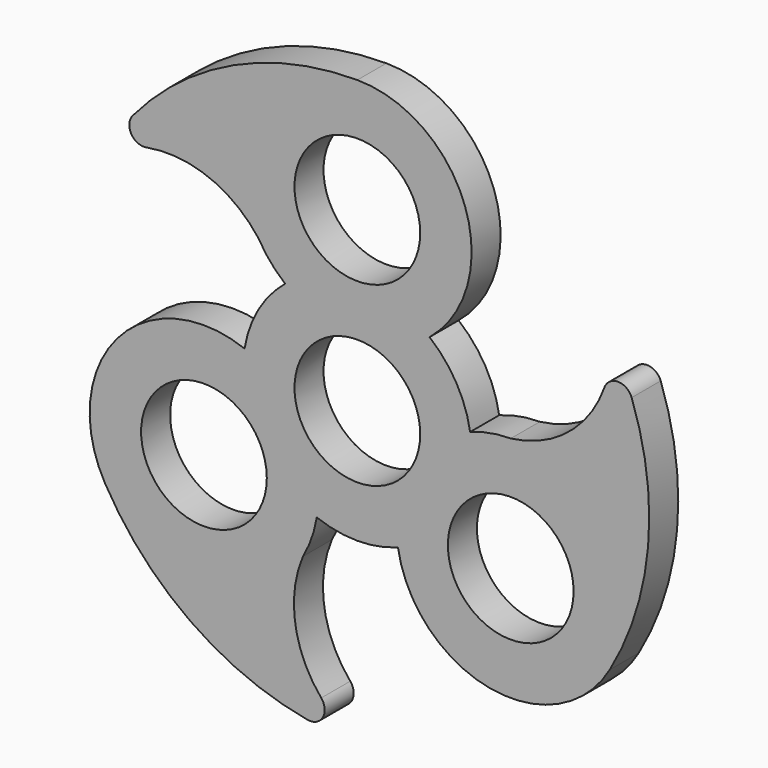
from build123d import *

# Parameters (mm, degrees)
F1_R     = 11
F2_DEPTH = 3.175
F3_COUNT = 3


# Not quite as in the source:
# - a length typed as a fraction of an inch, garbled in the dataset ("3 / 203.2 mm" for 3/8 in), is restored
# - a feature names something its author has since deleted; it is built from what else it names


with BuildPart() as f2:
    # F1 (on Front) → F2 (new body, symmetric)
    with BuildSketch(Plane.XZ):
        with BuildLine():
            ThreePointArc((-17.3205080757, 21), (-15.23019686, 18.0369330942), (-12.6392246598, 15.5))
            ThreePointArc((-12.6392246598, 15.5), (0, -20), (12.6392246598, 15.5))
            ThreePointArc((12.6392246598, 15.5), (18.8414436814, 37.7082039325), (0, 51))
            ThreePointArc((0, 51), (-17.3205080757, 41), (-17.3205080757, 21))
        make_face()
        Circle(F1_R, mode=Mode.SUBTRACT)
        with Locations((0, 31)):
            Circle(F1_R, mode=Mode.SUBTRACT)
        with BuildLine():
            ThreePointArc((-36.9078890595, 28.6072001494), (-26.0346725644, 27.5832150042), (-17.3205080757, 21))
            ThreePointArc((-17.3205080757, 21), (-17.3205080757, 41), (0, 51))
            ThreePointArc((0, 51), (-21.6847928721, 46.2353229864), (-39.3138154874, 32.7390290291))
            ThreePointArc((-39.3138154874, 32.7390290291), (-39.5642297797, 29.8268260681), (-36.9078890595, 28.6072001494))
        make_face()
    extrude(amount=F2_DEPTH, both=True)

    # F3: F2 ×3 about axis
    f3_axis = Axis((0, -3.175, 0), (0, -1, 0))


with BuildPart() as f2_1:
    add(f2.part)
    for i in range(1, F3_COUNT):
        add(f2.part.rotate(f3_axis, i * 360 / F3_COUNT))


solid = f2_1.part
